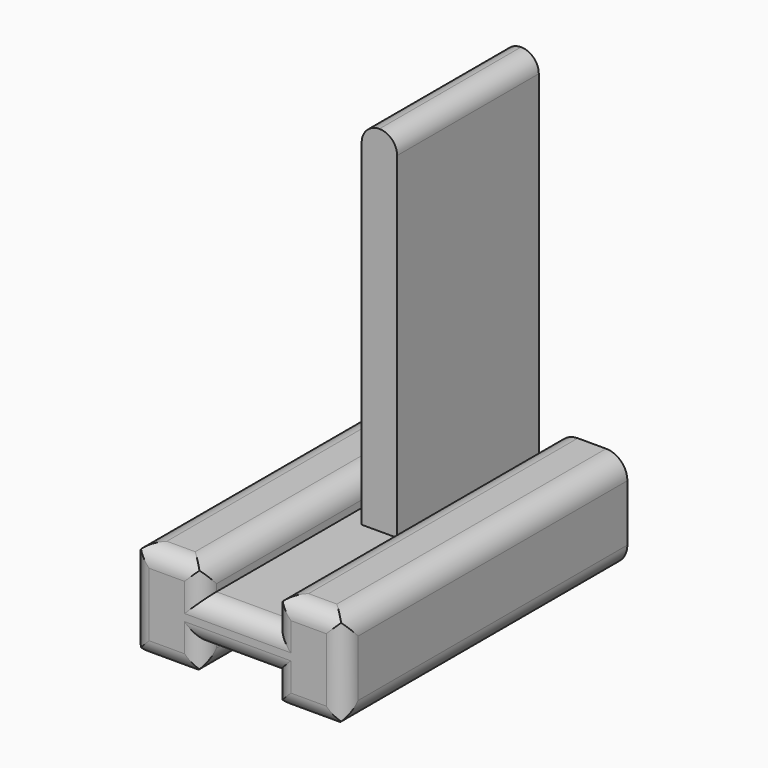
from build123d import *

# Parameters (mm, degrees)
F0_W        = 1.5
F0_H        = 1.2
F0_W_2      = 0.5
F0_W_3      = 1
F1_DEPTH    = 10
F0_H_2      = 10
F0_H_3      = 0.8
F2_DEPTH    = 5
F3_R        = 0.49999
F4_R        = 0.5
F5_T1_DEPTH = 12.5


# Not quite as in the source:
# - a fillet or chamfer that OpenCascade refuses, or shapes differently, is made with other operations: its cross-section is extruded or revolved along the edge and cut away or added
# - a fillet or chamfer is up to 0.001 mm smaller than in the source, because OpenCascade refuses the exact size


with BuildPart() as f1:
    # F0 (on Front) → F1 (new body)
    with BuildSketch(Plane.XZ):
        Polygon((1, 0.6), (2.5, 0.6), (2.5, -0.6), (1, -0.6), (1, -1.4), (3, -1.4), (3, 1.4), (1, 1.4), align=None)
        Polygon((-2.5, 0.6), (-1, 0.6), (-1, 1.4), (-3, 1.4), (-3, -1.4), (-1, -1.4), (-1, -0.6), (-2.5, -0.6), align=None)
        with Locations((1.75, 0)):
            Rectangle(F0_W, F0_H)
        with Locations((0.75, 0)):
            Rectangle(F0_W_2, F0_H)
        with Locations((-0.75, 0)):
            Rectangle(F0_W_2, F0_H)
        with Locations((-1.75, 0)):
            Rectangle(F0_W, F0_H)
        Rectangle(F0_W_3, F0_H)
    extrude(amount=F1_DEPTH)

    # F0 (on Front) → F2 (join)
    with BuildSketch(Plane.XZ):
        with Locations((0, 5.6)):
            Rectangle(F0_W_3, F0_H_2)
        with Locations((0, -1)):
            Rectangle(F0_W_3, F0_H_3)
    extrude(amount=F2_DEPTH)

    # F3 (radius 0.5 in the source; OpenCascade refuses exactly that, so slightly less here)
    f3_edges = [f1.edges().sort_by_distance(p)[0] for p in [
        (0.5, -2.5, 10.6),
        (-0.5, -2.5, 10.6),
    ]]
    fillet(f3_edges, radius=F3_R)

    # F4
    f4_edges = [f1.edges().sort_by_distance(p)[0] for p in [
        (2, -10, -1.4),
        (3, -10, 0),
        (2, -10, 1.4),
        (1, -10, 1),
        (0, -10, 0.6),
        (-1, -10, 1),
        (-2, -10, 1.4),
        (-3, -10, 0),
        (-2, -10, -1.4),
        (-1, -10, -1),
        (0, -10, -0.6),
        (1, -10, -1),
    ]]
    fillet(f4_edges, radius=F4_R)

    # F5: fillet of radius 0.6 on 8 edges, made by hand

    # F5_s2 → F5_t1 (cut)
    with BuildSketch(Plane.XZ.offset(-1.5)):
        with BuildLine():
            ThreePointArc((-2.4, 1.4), (-2.8242640687, 1.2242640687), (-3, 0.8))
            Line((-3, 0.8), (-3, 1.4))
            Line((-3, 1.4), (-2.4, 1.4))
        make_face()
        with BuildLine():
            ThreePointArc((-1, 0.8), (-1.1757359313, 1.2242640687), (-1.6, 1.4))
            Line((-1.6, 1.4), (-1, 1.4))
            Line((-1, 1.4), (-1, 0.8))
        make_face()
        with BuildLine():
            ThreePointArc((1, 0.8), (1.1757359313, 1.2242640687), (1.6, 1.4))
            Line((1.6, 1.4), (1, 1.4))
            Line((1, 1.4), (1, 0.8))
        make_face()
        with BuildLine():
            ThreePointArc((2.4, 1.4), (2.8242640687, 1.2242640687), (3, 0.8))
            Line((3, 0.8), (3, 1.4))
            Line((3, 1.4), (2.4, 1.4))
        make_face()
        with BuildLine():
            ThreePointArc((-3, -0.8), (-2.8242640687, -1.2242640687), (-2.4, -1.4))
            Line((-2.4, -1.4), (-3, -1.4))
            Line((-3, -1.4), (-3, -0.8))
        make_face()
        with BuildLine():
            ThreePointArc((-1.6, -1.4), (-1.1757359313, -1.2242640687), (-1, -0.8))
            Line((-1, -0.8), (-1, -1.4))
            Line((-1, -1.4), (-1.6, -1.4))
        make_face()
        with BuildLine():
            ThreePointArc((1.6, -1.4), (1.1757359313, -1.2242640687), (1, -0.8))
            Line((1, -0.8), (1, -1.4))
            Line((1, -1.4), (1.6, -1.4))
        make_face()
        with BuildLine():
            ThreePointArc((3, -0.8), (2.8242640687, -1.2242640687), (2.4, -1.4))
            Line((2.4, -1.4), (3, -1.4))
            Line((3, -1.4), (3, -0.8))
        make_face()
    extrude(amount=F5_T1_DEPTH, mode=Mode.SUBTRACT)


solid = f1.part
